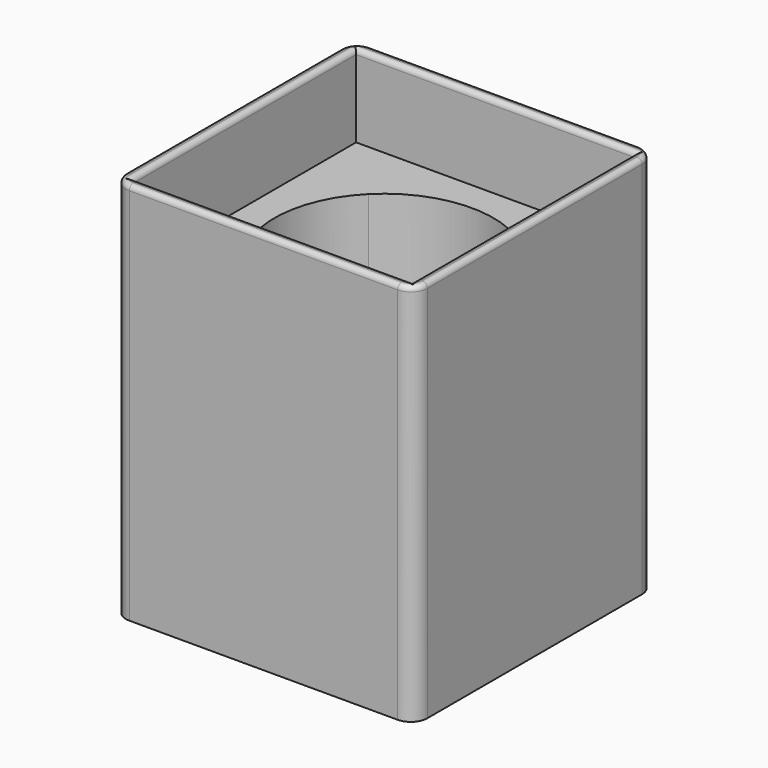
from build123d import *

# Parameters (mm, degrees)
F0_W         = 51
F0_H         = 51
F1_DEPTH     = 55
F2_DEPTH     = 70
F4_DEPTH     = 50
F5_DEPTH     = 100
F6_R         = 3
F7_T1_DEPTH  = 51
F7_T3_DEPTH  = 51
F7_T5_DEPTH  = 49
F7_T7_DEPTH  = 49
F7_T10_ANGLE = 90
F7_T12_ANGLE = 90
F7_T14_ANGLE = 90
F7_T16_ANGLE = 90
F7_T21_DEPTH = 53.25
F7_T25_DEPTH = 53.25
F7_T32_DEPTH = 53.25
F7_T36_DEPTH = 53.25
F7_T43_DEPTH = 53.25
F7_T47_DEPTH = 53.25
F7_T54_DEPTH = 53.25
F7_T58_DEPTH = 53.25


# Not quite as in the source:
# - a fillet or chamfer that OpenCascade refuses, or shapes differently, is made with other operations: its cross-section is extruded or revolved along the edge and cut away or added


with BuildPart() as f1:
    # F0 (on Top) → F1 (new body)
    with BuildSketch(Plane.XY):
        with Locations((-25.5, 25.5)):
            Rectangle(F0_W, F0_H)
    extrude(amount=F1_DEPTH)

    # F0 (on Top) → F2 (join)
    with BuildSketch(Plane.XY):
        Polygon((-51, -2), (-51, 0), (-51, 51), (0, 51), (2, 51), (2, 53), (-53, 53), (-53, -2), align=None)
        Polygon((0, 51), (0, 0), (-51, 0), (-51, -2), (0, -2), (2, -2), (2, 51), align=None)
    extrude(amount=F2_DEPTH)

    # F3 (on face) → F4 (cut)
    with BuildSketch(Plane.XY.offset(55)):
        with BuildLine():
            Line((-26.9142135624, 26.9142135624), (-39.6421356237, 39.6421356237))
            ThreePointArc((-39.6421356237, 39.6421356237), (-45.5, 25.5), (-39.6421356237, 11.3578643763))
            Line((-39.6421356237, 11.3578643763), (-26.9142135624, 24.0857864376))
            ThreePointArc((-26.9142135624, 24.0857864376), (-27.5, 25.5), (-26.9142135624, 26.9142135624))
        make_face()
        with BuildLine():
            Line((-24.0857864376, 26.9142135624), (-25.5, 25.5))
            Line((-25.5, 25.5), (-24.0857864376, 24.0857864376))
            ThreePointArc((-24.0857864376, 24.0857864376), (-23.652240935, 24.7346331353), (-23.5, 25.5))
            ThreePointArc((-23.5, 25.5), (-23.652240935, 26.2653668647), (-24.0857864376, 26.9142135624))
        make_face()
        with BuildLine():
            Line((-24.0857864376, 24.0857864376), (-25.5, 25.5))
            Line((-25.5, 25.5), (-26.9142135624, 24.0857864376))
            ThreePointArc((-26.9142135624, 24.0857864376), (-25.5, 23.5), (-24.0857864376, 24.0857864376))
        make_face()
        with BuildLine():
            ThreePointArc((-11.3578643763, 39.6421356237), (-25.5, 45.5), (-39.6421356237, 39.6421356237))
            Line((-39.6421356237, 39.6421356237), (-26.9142135624, 26.9142135624))
            ThreePointArc((-26.9142135624, 26.9142135624), (-25.5, 27.5), (-24.0857864376, 26.9142135624))
            Line((-24.0857864376, 26.9142135624), (-11.3578643763, 39.6421356237))
        make_face()
        with BuildLine():
            Line((-25.5, 25.5), (-26.9142135624, 26.9142135624))
            ThreePointArc((-26.9142135624, 26.9142135624), (-27.5, 25.5), (-26.9142135624, 24.0857864376))
            Line((-26.9142135624, 24.0857864376), (-25.5, 25.5))
        make_face()
        with BuildLine():
            ThreePointArc((-5.5, 25.5), (-7.0224093498, 33.1536686473), (-11.3578643763, 39.6421356237))
            Line((-11.3578643763, 39.6421356237), (-24.0857864376, 26.9142135624))
            ThreePointArc((-24.0857864376, 26.9142135624), (-23.652240935, 26.2653668647), (-23.5, 25.5))
            ThreePointArc((-23.5, 25.5), (-23.652240935, 24.7346331353), (-24.0857864376, 24.0857864376))
            Line((-24.0857864376, 24.0857864376), (-11.3578643763, 11.3578643763))
            ThreePointArc((-11.3578643763, 11.3578643763), (-7.0224093498, 17.8463313527), (-5.5, 25.5))
        make_face()
        with BuildLine():
            Line((-26.9142135624, 24.0857864376), (-39.6421356237, 11.3578643763))
            ThreePointArc((-39.6421356237, 11.3578643763), (-25.5, 5.5), (-11.3578643763, 11.3578643763))
            Line((-11.3578643763, 11.3578643763), (-24.0857864376, 24.0857864376))
            ThreePointArc((-24.0857864376, 24.0857864376), (-25.5, 23.5), (-26.9142135624, 24.0857864376))
        make_face()
        with BuildLine():
            ThreePointArc((-24.0857864376, 26.9142135624), (-25.5, 27.5), (-26.9142135624, 26.9142135624))
            Line((-26.9142135624, 26.9142135624), (-25.5, 25.5))
            Line((-25.5, 25.5), (-24.0857864376, 26.9142135624))
        make_face()
    extrude(amount=-F4_DEPTH, mode=Mode.SUBTRACT)

    # F3 (on face) → F5 (cut)
    with BuildSketch(Plane.XY.offset(55)):
        with BuildLine():
            ThreePointArc((-24.0857864376, 26.9142135624), (-25.5, 27.5), (-26.9142135624, 26.9142135624))
            Line((-26.9142135624, 26.9142135624), (-25.5, 25.5))
            Line((-25.5, 25.5), (-24.0857864376, 26.9142135624))
        make_face()
        with BuildLine():
            Line((-24.0857864376, 26.9142135624), (-25.5, 25.5))
            Line((-25.5, 25.5), (-24.0857864376, 24.0857864376))
            ThreePointArc((-24.0857864376, 24.0857864376), (-23.652240935, 24.7346331353), (-23.5, 25.5))
            ThreePointArc((-23.5, 25.5), (-23.652240935, 26.2653668647), (-24.0857864376, 26.9142135624))
        make_face()
        with BuildLine():
            Line((-24.0857864376, 24.0857864376), (-25.5, 25.5))
            Line((-25.5, 25.5), (-26.9142135624, 24.0857864376))
            ThreePointArc((-26.9142135624, 24.0857864376), (-25.5, 23.5), (-24.0857864376, 24.0857864376))
        make_face()
        with BuildLine():
            Line((-25.5, 25.5), (-26.9142135624, 26.9142135624))
            ThreePointArc((-26.9142135624, 26.9142135624), (-27.5, 25.5), (-26.9142135624, 24.0857864376))
            Line((-26.9142135624, 24.0857864376), (-25.5, 25.5))
        make_face()
    extrude(amount=-F5_DEPTH, mode=Mode.SUBTRACT)

    # F6
    f6_edges = [f1.edges().sort_by_distance(p)[0] for p in [
        (2, 53, 35),
        (-53, 53, 35),
        (-53, -2, 35),
        (2, -2, 35),
    ]]
    fillet(f6_edges, radius=F6_R)

    # F7: fillet of radius 0.9 on 5 edges, made by hand

    # F7_s2 → F7_t1 (cut)
    with BuildSketch(Plane.XZ.offset(-51)):
        with BuildLine():
            ThreePointArc((0.9, 70), (0.2636038969, 69.7363961031), (0, 69.1))
            Line((0, 69.1), (0, 70))
            Line((0, 70), (0.9, 70))
        make_face()
        with BuildLine():
            ThreePointArc((-51.9, 70), (-51.2636038969, 69.7363961031), (-51, 69.1))
            Line((-51, 69.1), (-51, 70))
            Line((-51, 70), (-51.9, 70))
        make_face()
    extrude(amount=F7_T1_DEPTH, mode=Mode.SUBTRACT)

    # F7_s4 → F7_t3 (cut)
    with BuildSketch(Plane.YZ.offset(-51)):
        with BuildLine():
            ThreePointArc((51.9, 70), (51.2636038969, 69.7363961031), (51, 69.1))
            Line((51, 69.1), (51, 70))
            Line((51, 70), (51.9, 70))
        make_face()
        with BuildLine():
            ThreePointArc((-0.9, 70), (-0.2636038969, 69.7363961031), (0, 69.1))
            Line((0, 69.1), (0, 70))
            Line((0, 70), (-0.9, 70))
        make_face()
    extrude(amount=F7_T3_DEPTH, mode=Mode.SUBTRACT)

    # F7_s6 → F7_t5 (cut)
    with BuildSketch(Plane.YZ.offset(-50)):
        with BuildLine():
            ThreePointArc((-2, 69.1), (-1.7363961031, 69.7363961031), (-1.1, 70))
            Line((-1.1, 70), (-2, 70))
            Line((-2, 70), (-2, 69.1))
        make_face()
        with BuildLine():
            ThreePointArc((53, 69.1), (52.7363961031, 69.7363961031), (52.1, 70))
            Line((52.1, 70), (53, 70))
            Line((53, 70), (53, 69.1))
        make_face()
    extrude(amount=F7_T5_DEPTH, mode=Mode.SUBTRACT)

    # F7_s8 → F7_t7 (cut)
    with BuildSketch(Plane.XZ.offset(-50)):
        with BuildLine():
            ThreePointArc((2, 69.1), (1.7363961031, 69.7363961031), (1.1, 70))
            Line((1.1, 70), (2, 70))
            Line((2, 70), (2, 69.1))
        make_face()
        with BuildLine():
            ThreePointArc((-53, 69.1), (-52.7363961031, 69.7363961031), (-52.1, 70))
            Line((-52.1, 70), (-53, 70))
            Line((-53, 70), (-53, 69.1))
        make_face()
    extrude(amount=F7_T7_DEPTH, mode=Mode.SUBTRACT)

    # F7_s9 → F7_t10 (revolve, cut)
    with BuildSketch(Plane.XZ.offset(-1)):
        with BuildLine():
            ThreePointArc((-53, 69.1), (-52.7363961031, 69.7363961031), (-52.1, 70))
            Line((-52.1, 70), (-53, 70))
            Line((-53, 70), (-53, 69.1))
        make_face()
    revolve(axis=Axis((-50, 1, 70), (0, 0, 1)), revolution_arc=F7_T10_ANGLE, mode=Mode.SUBTRACT)

    # F7_s11 → F7_t12 (revolve, cut)
    with BuildSketch(Plane.XZ.offset(-1)):
        with BuildLine():
            ThreePointArc((2, 69.1), (1.7363961031, 69.7363961031), (1.1, 70))
            Line((1.1, 70), (2, 70))
            Line((2, 70), (2, 69.1))
        make_face()
    revolve(axis=Axis((-1, 1, 70), (0, 0, -1)), revolution_arc=F7_T12_ANGLE, mode=Mode.SUBTRACT)

    # F7_s13 → F7_t14 (revolve, cut)
    with BuildSketch(Plane.YZ.offset(-1)):
        with BuildLine():
            ThreePointArc((53, 69.1), (52.7363961031, 69.7363961031), (52.1, 70))
            Line((52.1, 70), (53, 70))
            Line((53, 70), (53, 69.1))
        make_face()
    revolve(axis=Axis((-1, 50, 70), (0, 0, -1)), revolution_arc=F7_T14_ANGLE, mode=Mode.SUBTRACT)

    # F7_s15 → F7_t16 (revolve, cut)
    with BuildSketch(Plane.YZ.offset(-50)):
        with BuildLine():
            ThreePointArc((53, 69.1), (52.7363961031, 69.7363961031), (52.1, 70))
            Line((52.1, 70), (53, 70))
            Line((53, 70), (53, 69.1))
        make_face()
    revolve(axis=Axis((-50, 50, 70), (0, 0, 1)), revolution_arc=F7_T16_ANGLE, mode=Mode.SUBTRACT)


with BuildPart() as f7_tool19:
    # F7_s20 → F7_t21 (new body)
    with BuildSketch(Plane.YZ.offset(-51)):
        with BuildLine():
            ThreePointArc((51.9, 70), (51.2636038969, 69.7363961031), (51, 69.1))
            Line((51, 69.1), (51, 70))
            Line((51, 70), (51.9, 70))
        make_face()
    extrude(amount=F7_T21_DEPTH)

    split(bisect_by=Plane.YZ, keep=Keep.TOP)


with BuildPart() as f7_tool23:
    # F7_s24 → F7_t25 (new body)
    with BuildSketch(Plane.XZ.offset(-53.25)):
        with BuildLine():
            ThreePointArc((0.9, 70), (0.2636038969, 69.7363961031), (0, 69.1))
            Line((0, 69.1), (0, 70))
            Line((0, 70), (0.9, 70))
        make_face()
    extrude(amount=F7_T25_DEPTH)

    split(bisect_by=Plane.XZ.offset(-51), keep=Keep.BOTTOM)


with BuildPart() as f7_tool19_1:
    add(f7_tool19.part)

    # F7_t27: intersect F7_tool23
    add(f7_tool23.part, mode=Mode.INTERSECT)


with BuildPart() as f1_1:
    add(f1.part)

    # F7_t17: cut F7_tool19
    add(f7_tool19_1.part, mode=Mode.SUBTRACT)


with BuildPart() as f7_tool30:
    # F7_s31 → F7_t32 (new body)
    with BuildSketch(Plane.XZ.offset(-51)):
        with BuildLine():
            ThreePointArc((0.9, 70), (0.2636038969, 69.7363961031), (0, 69.1))
            Line((0, 69.1), (0, 70))
            Line((0, 70), (0.9, 70))
        make_face()
    extrude(amount=F7_T32_DEPTH)

    split(bisect_by=Plane.XZ, keep=Keep.TOP)


with BuildPart() as f7_tool34:
    # F7_s35 → F7_t36 (new body)
    with BuildSketch(Plane.YZ.offset(2.25)):
        with BuildLine():
            ThreePointArc((-0.9, 70), (-0.2636038969, 69.7363961031), (0, 69.1))
            Line((0, 69.1), (0, 70))
            Line((0, 70), (-0.9, 70))
        make_face()
    extrude(amount=-F7_T36_DEPTH)

    split(bisect_by=Plane.YZ, keep=Keep.TOP)


with BuildPart() as f7_tool30_1:
    add(f7_tool30.part)

    # F7_t38: intersect F7_tool34
    add(f7_tool34.part, mode=Mode.INTERSECT)


with BuildPart() as f1_2:
    add(f1_1.part)

    # F7_t28: cut F7_tool30
    add(f7_tool30_1.part, mode=Mode.SUBTRACT)


with BuildPart() as f7_tool41:
    # F7_s42 → F7_t43 (new body)
    with BuildSketch(Plane.XZ):
        with BuildLine():
            ThreePointArc((-51.9, 70), (-51.2636038969, 69.7363961031), (-51, 69.1))
            Line((-51, 69.1), (-51, 70))
            Line((-51, 70), (-51.9, 70))
        make_face()
    extrude(amount=-F7_T43_DEPTH)

    split(bisect_by=Plane.XZ.offset(-51), keep=Keep.BOTTOM)


with BuildPart() as f7_tool45:
    # F7_s46 → F7_t47 (new body)
    with BuildSketch(Plane.YZ.offset(-53.25)):
        with BuildLine():
            ThreePointArc((51.9, 70), (51.2636038969, 69.7363961031), (51, 69.1))
            Line((51, 69.1), (51, 70))
            Line((51, 70), (51.9, 70))
        make_face()
    extrude(amount=F7_T47_DEPTH)

    split(bisect_by=Plane.YZ.offset(-51), keep=Keep.BOTTOM)


with BuildPart() as f7_tool41_1:
    add(f7_tool41.part)

    # F7_t49: intersect F7_tool45
    add(f7_tool45.part, mode=Mode.INTERSECT)


with BuildPart() as f1_3:
    add(f1_2.part)

    # F7_t39: cut F7_tool41
    add(f7_tool41_1.part, mode=Mode.SUBTRACT)


with BuildPart() as f7_tool52:
    # F7_s53 → F7_t54 (new body)
    with BuildSketch(Plane.XZ.offset(2.25)):
        with BuildLine():
            ThreePointArc((-51.9, 70), (-51.2636038969, 69.7363961031), (-51, 69.1))
            Line((-51, 69.1), (-51, 70))
            Line((-51, 70), (-51.9, 70))
        make_face()
    extrude(amount=-F7_T54_DEPTH)

    split(bisect_by=Plane.XZ, keep=Keep.TOP)


with BuildPart() as f7_tool56:
    # F7_s57 → F7_t58 (new body)
    with BuildSketch(Plane.YZ):
        with BuildLine():
            ThreePointArc((-0.9, 70), (-0.2636038969, 69.7363961031), (0, 69.1))
            Line((0, 69.1), (0, 70))
            Line((0, 70), (-0.9, 70))
        make_face()
    extrude(amount=-F7_T58_DEPTH)

    split(bisect_by=Plane.YZ.offset(-51), keep=Keep.BOTTOM)


with BuildPart() as f7_tool52_1:
    add(f7_tool52.part)

    # F7_t60: intersect F7_tool56
    add(f7_tool56.part, mode=Mode.INTERSECT)


with BuildPart() as f1_4:
    add(f1_3.part)

    # F7_t50: cut F7_tool52
    add(f7_tool52_1.part, mode=Mode.SUBTRACT)


solid = f1_4.part
